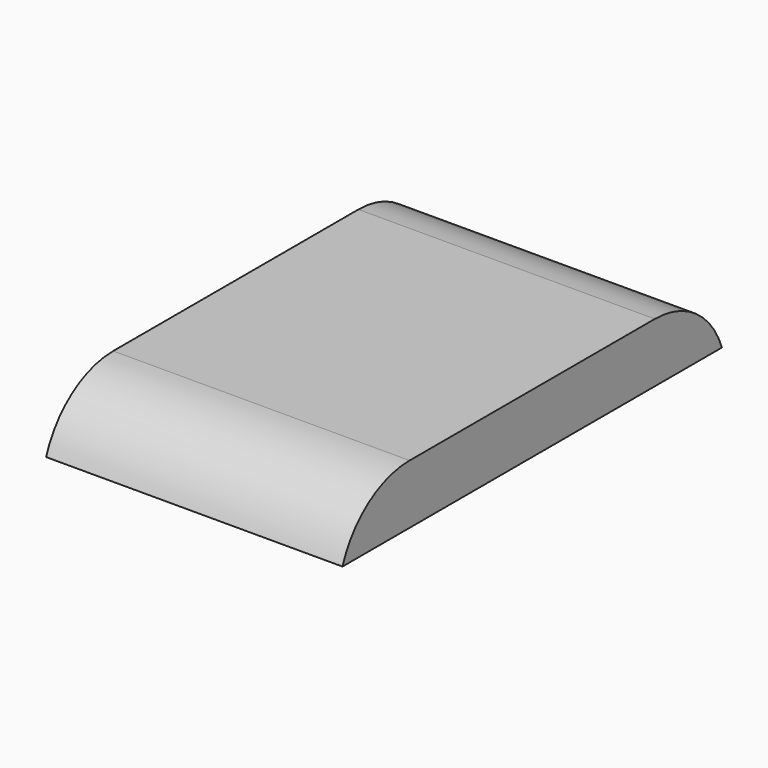
from build123d import *

# Parameters (mm, degrees)
F0_W        = 254
F0_H        = 406.4
F1_DEPTH    = 25.4
F2_T1_DEPTH = 613.2102448428


# Not quite as in the source:
# - a fillet or chamfer that OpenCascade refuses, or shapes differently, is made with other operations: its cross-section is extruded or revolved along the edge and cut away or added


with BuildPart() as f1:
    # F0 (on Top) → F1 (new body, symmetric)
    with BuildSketch(Plane.XY):
        Rectangle(F0_W, F0_H)
    extrude(amount=F1_DEPTH, both=True)

    # F2: fillet of radius 76.2 on 2 edges, made by hand

    # F2_s2 → F2_t1 (cut)
    with BuildSketch(Plane.YZ.offset(-306.6051224214)):
        with BuildLine():
            ThreePointArc((203.2, -25.4), (175.3520415437, 11.4170394667), (131.3579510314, 25.4))
            Line((131.3579510314, 25.4), (203.2, 25.4))
            Line((203.2, 25.4), (203.2, -25.4))
        make_face()
        with BuildLine():
            ThreePointArc((-203.2, -25.4), (-175.3520415437, 11.4170394667), (-131.3579510314, 25.4))
            Line((-131.3579510314, 25.4), (-203.2, 25.4))
            Line((-203.2, 25.4), (-203.2, -25.4))
        make_face()
    extrude(amount=F2_T1_DEPTH, mode=Mode.SUBTRACT)


solid = f1.part
